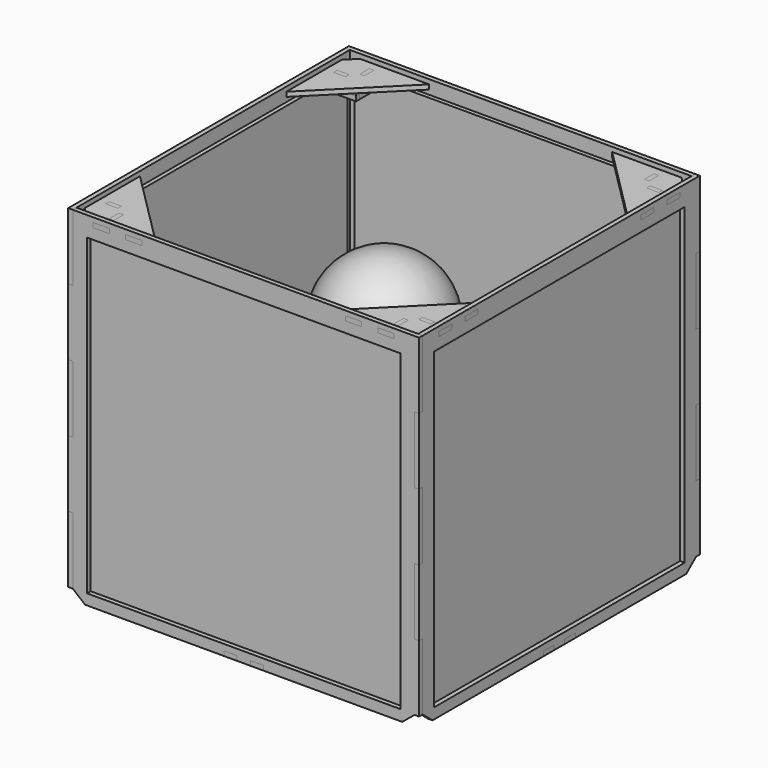
from build123d import *

# Parameters (mm, degrees)
F3_R      = 16
F3_R_2    = 15
F4_DEPTH  = 2.25
F5_W      = 2.25
F5_H      = 6.9285714286
F6_DEPTH  = 38
F7_DEPTH  = 2.25
F8_W      = 2.25
F8_H      = 6.6
F8_W_2    = 6.5
F8_H_2    = 2.25
F9_DEPTH  = 2.25
F11_W     = 160
F11_H     = 160
F12_DEPTH = 2
F13_W     = 154
F13_H     = 154
F13_W_2   = 8
F13_H_2   = 2.25
F14_DEPTH = 2.25
F15_W     = 6
F15_H     = 2.25
F15_W_2   = 2.25
F15_H_2   = 6
F16_DEPTH = 2.25
F18_DEPTH = 2.25
F20_DEPTH = 2.25
F21_W     = 2.25
F21_H     = 6.5
F21_W_2   = 4
F21_H_2   = 2.25
F22_DEPTH = 2.25
F24_DEPTH = 2.25
F25_COUNT = 4


with BuildPart() as f2:
    # F1 (on Front) → F2 (revolve)
    with BuildSketch(Plane.XZ):
        with BuildLine():
            Line((0, 143), (0, 10))
            Line((0, 10), (10, 10))
            Line((10, 10), (11.5, 20))
            Line((11.5, 20), (12.5, 25))
            Line((12.5, 25), (12.5, 36))
            Line((12.5, 36), (16, 36))
            Line((16, 36), (16, 38))
            Line((16, 38), (14, 38))
            Line((14, 38), (14, 40.25))
            Line((14, 40.25), (17.5, 40.25))
            Line((17.5, 40.25), (15, 48.25))
            Line((15, 48.25), (14, 48.25))
            Line((14, 48.25), (14, 63))
            Line((14, 63), (20, 72))
            Line((20, 72), (20, 85))
            Line((20, 85), (24, 95))
            ThreePointArc((24, 95), (26.83281573, 126.416407865), (0, 143))
        make_face()
    revolve(axis=Axis((0, 0, 76.5), (0, 0, -1)))


with BuildPart() as f4:
    # F3 (on face) → F4 (new body)
    with BuildSketch(Plane.XY.offset(38)):
        Polygon((-10.3928571429, 22), (-17.3214285714, 22), (-17.3214285714, 24.25), (-24.25, 24.25), (-24.25, 17.3214285714), (-22, 17.3214285714), (-22, 10.3928571429), (-24.25, 10.3928571429), (-24.25, 3.4642857143), (-22, 3.4642857143), (-22, -3.4642857143), (-24.25, -3.4642857143), (-24.25, -10.3928571429), (-22, -10.3928571429), (-22, -17.3214285714), (-24.25, -17.3214285714), (-24.25, -24.25), (-17.3214285714, -24.25), (-17.3214285714, -22), (-10.3928571429, -22), (-10.3928571429, -24.25), (-3.4642857143, -24.25), (-3.4642857143, -22), (3.4642857143, -22), (3.4642857143, -24.25), (10.3928571429, -24.25), (10.3928571429, -22), (17.3214285714, -22), (17.3214285714, -24.25), (24.25, -24.25), (24.25, -17.3214285714), (22, -17.3214285714), (22, -10.3928571429), (24.25, -10.3928571429), (24.25, -3.4642857143), (22, -3.4642857143), (22, 3.4642857143), (24.25, 3.4642857143), (24.25, 10.3928571429), (22, 10.3928571429), (22, 17.3214285714), (24.25, 17.3214285714), (24.25, 24.25), (17.3214285714, 24.25), (17.3214285714, 22), (10.3928571429, 22), (10.3928571429, 24.25), (3.4642857143, 24.25), (3.4642857143, 22), (-3.4642857143, 22), (-3.4642857143, 24.25), (-10.3928571429, 24.25), align=None)
        Circle(F3_R, mode=Mode.SUBTRACT)
        Circle(F3_R)
        Circle(F3_R_2, mode=Mode.SUBTRACT)
    extrude(amount=F4_DEPTH)


with BuildPart() as f6:
    # F5 (on face) → F6 (new body, through all)
    with BuildSketch(Plane(origin=(0, 0, 38), x_dir=(1, 0, 0), z_dir=(0, 0, -1))):
        with Locations((-23.125, 20.7857142857)):
            Rectangle(F5_W, F5_H)
        with Locations((-23.125, 13.8571428571)):
            Rectangle(F5_W, F5_H)
        with Locations((-23.125, 6.9285714286)):
            Rectangle(F5_W, F5_H)
        with Locations((-23.125, 0)):
            Rectangle(F5_W, F5_H)
        with Locations((-23.125, -6.9285714286)):
            Rectangle(F5_W, F5_H)
        with Locations((-23.125, -13.8571428571)):
            Rectangle(F5_W, F5_H)
        with Locations((-23.125, -20.7857142857)):
            Rectangle(F5_W, F5_H)
    extrude(amount=F6_DEPTH)

    # F5 (on face) → F7 (join, through all)
    with BuildSketch(Plane(origin=(0, 0, 38), x_dir=(1, 0, 0), z_dir=(0, 0, -1))):
        with Locations((-23.125, -13.8571428571)):
            Rectangle(F5_W, F5_H)
        with Locations((-23.125, 0)):
            Rectangle(F5_W, F5_H)
        with Locations((-23.125, 13.8571428571)):
            Rectangle(F5_W, F5_H)
    extrude(amount=-F7_DEPTH)

    # F8 (on face) → F9 (cut, through all)
    with BuildSketch(Plane(origin=(-24.25, 0, 0), x_dir=(0, -1, 0), z_dir=(-1, 0, 0))):
        Polygon((-24.25, 5), (-24.25, 0), (-9.75, 0), (-9.75, 2.25), (-16.25, 2.25), (-16.25, 5), align=None)
        Polygon((9.75, 0), (24.25, 0), (24.25, 5), (24.25, 11.6), (22, 11.6), (22, 5), (16.25, 5), (16.25, 2.25), (9.75, 2.25), align=None)
        with Locations((-23.125, 28.1)):
            Rectangle(F8_W, F8_H)
        with Locations((-23.125, 14.9)):
            Rectangle(F8_W, F8_H)
        with Locations((23.125, 34.7)):
            Rectangle(F8_W, F8_H)
        with Locations((23.125, 21.5)):
            Rectangle(F8_W, F8_H)
        with Locations((0, 1.125)):
            Rectangle(F8_W_2, F8_H_2)
    extrude(amount=-F9_DEPTH, mode=Mode.SUBTRACT)


with BuildPart() as f12:
    # F11 (on offset) → F12 (new body)
    with BuildSketch(Plane.YZ.offset(-82)):
        with Locations((0, 82.25)):
            Rectangle(F11_W, F11_H)
    extrude(amount=-F12_DEPTH)


with BuildPart() as f14:
    # F13 (on face) → F14 (new body)
    with BuildSketch(Plane(origin=(-84, 0, 0), x_dir=(0, -1, 0), z_dir=(-1, 0, 0))):
        Polygon((-84, 136.2), (-86.25, 136.2), (-86.25, 103.4), (-84, 103.4), (-84, 70.6), (-86.25, 70.6), (-86.25, 37.8), (-84, 37.8), (-84, 5), (-78, 0), (-9.75, 0), (-9.75, 2.25), (-3.25, 2.25), (-3.25, 0), (3.25, 0), (3.25, 2.25), (9.75, 2.25), (9.75, 0), (78, 0), (84, 5), (86.25, 5), (86.25, 37.8), (84, 37.8), (84, 70.6), (86.25, 70.6), (86.25, 103.4), (84, 103.4), (84, 136.2), (86.25, 136.2), (86.25, 169), (-84, 169), align=None)
        with Locations((0, 82.25)):
            Rectangle(F13_W, F13_H, mode=Mode.SUBTRACT)
        with Locations((-70, 165.625)):
            Rectangle(F13_W_2, F13_H_2, mode=Mode.SUBTRACT)
        with Locations((-54, 165.625)):
            Rectangle(F13_W_2, F13_H_2, mode=Mode.SUBTRACT)
        with Locations((54, 165.625)):
            Rectangle(F13_W_2, F13_H_2, mode=Mode.SUBTRACT)
        with Locations((70, 165.625)):
            Rectangle(F13_W_2, F13_H_2, mode=Mode.SUBTRACT)
    extrude(amount=F14_DEPTH)


with BuildPart() as f16:
    # F15 (on face) → F16 (new body, through all)
    with BuildSketch(Plane.XY.offset(164.5)):
        Polygon((-84, 74), (-86.25, 74), (-86.25, 66), (-84, 66), (-84, 58), (-86.25, 58), (-86.25, 50), (-84, 50), (-84, 45), (-45, 84), (-50, 84), (-50, 86.25), (-58, 86.25), (-58, 84), (-66, 84), (-66, 86.25), (-74, 86.25), (-74, 84), (-79, 84), (-84, 79), align=None)
        with Locations((-77, 70)):
            Rectangle(F15_W, F15_H, mode=Mode.SUBTRACT)
        with Locations((-70, 77)):
            Rectangle(F15_W_2, F15_H_2, mode=Mode.SUBTRACT)
    extrude(amount=F16_DEPTH)


with BuildPart() as f18:
    # F17 (on face) → F18 (new body, through all)
    with BuildSketch(Plane.XZ.offset(-71.125)):
        Polygon((-74, 166.75), (-80, 166.75), (-80, 164.5), (-82, 164.5), (-82, 157.75), (-68.875, 157.75), (-68.875, 160), (-71.125, 160), (-71.125, 162.25), (-68.875, 162.25), (-68.875, 164.5), (-74, 164.5), align=None)
    extrude(amount=F18_DEPTH)


with BuildPart() as f20:
    # F19 (on face) → F20 (new body, through all)
    with BuildSketch(Plane.YZ.offset(-71.125)):
        Polygon((80, 164.5), (80, 166.75), (74, 166.75), (74, 164.5), (71.125, 164.5), (71.125, 162.25), (68.8749999992, 162.25), (68.875, 160), (71.1249999993, 160), (71.125, 157.75), (82, 157.75), (82, 164.5), align=None)
    extrude(amount=F20_DEPTH)


with BuildPart() as f22:
    # F21 (on Top) → F22 (new body)
    with BuildSketch(Plane.XY):
        Polygon((-22, 16.25), (-84, 16.25), (-84, 9.75), (-86.25, 9.75), (-86.25, 3.25), (-84, 3.25), (-84, -3.25), (-86.25, -3.25), (-86.25, -9.75), (-84, -9.75), (-84, -16.25), (-22, -16.25), (-12.3743686708, -12.3743686708), (-10.2530483272, -10.2530483272), (-8.6620580695, -11.8440385849), (-4.0658639918, -7.2478445072), (-5.6568542495, -5.6568542495), (0, 0), (-5.6568542495, 5.6568542495), (-7.2478445072, 4.0658639918), (-11.8440385849, 8.6620580695), (-10.2530483272, 10.2530483272), (-12.3743686708, 12.3743686708), align=None)
        with Locations((-23.125, -6.5)):
            Rectangle(F21_W, F21_H, mode=Mode.SUBTRACT)
        with Locations((-76, 0)):
            Rectangle(F21_W_2, F21_H_2, mode=Mode.SUBTRACT)
        with Locations((-68, 0)):
            Rectangle(F21_W_2, F21_H_2, mode=Mode.SUBTRACT)
        with Locations((-23.125, 6.5)):
            Rectangle(F21_W, F21_H, mode=Mode.SUBTRACT)
    extrude(amount=F22_DEPTH)


with BuildPart() as f24:
    # F23 (on face) → F24 (new body, through all)
    with BuildSketch(Plane.XZ.offset(-1.125)):
        Polygon((-82, 2.25), (-78, 2.25), (-78, 0), (-74, 0), (-74, 2.25), (-70, 2.25), (-70, 0), (-66, 0), (-66, 2.25), (-62, 2.25), (-62, 6.25), (-82, 6.25), align=None)
    extrude(amount=F24_DEPTH)


with BuildPart() as f25_1:
    # F25: instance of F6
    add(f6.part.rotate(Axis((0, 0, 76.5), (0, 0, -1)), 1 * 360 / F25_COUNT))


with BuildPart() as f25_2:
    # F25: instance of F6
    add(f6.part.rotate(Axis((0, 0, 76.5), (0, 0, -1)), 2 * 360 / F25_COUNT))


with BuildPart() as f25_3:
    # F25: instance of F6
    add(f6.part.rotate(Axis((0, 0, 76.5), (0, 0, -1)), 3 * 360 / F25_COUNT))


with BuildPart() as f25_4:
    # F25: instance of F22
    add(f22.part.rotate(Axis((0, 0, 76.5), (0, 0, -1)), 1 * 360 / F25_COUNT))


with BuildPart() as f25_5:
    # F25: instance of F22
    add(f22.part.rotate(Axis((0, 0, 76.5), (0, 0, -1)), 2 * 360 / F25_COUNT))


with BuildPart() as f25_6:
    # F25: instance of F22
    add(f22.part.rotate(Axis((0, 0, 76.5), (0, 0, -1)), 3 * 360 / F25_COUNT))


with BuildPart() as f25_7:
    # F25: instance of F12
    add(f12.part.rotate(Axis((0, 0, 76.5), (0, 0, -1)), 1 * 360 / F25_COUNT))


with BuildPart() as f25_8:
    # F25: instance of F12
    add(f12.part.rotate(Axis((0, 0, 76.5), (0, 0, -1)), 2 * 360 / F25_COUNT))


with BuildPart() as f25_9:
    # F25: instance of F12
    add(f12.part.rotate(Axis((0, 0, 76.5), (0, 0, -1)), 3 * 360 / F25_COUNT))


with BuildPart() as f25_10:
    # F25: instance of F14
    add(f14.part.rotate(Axis((0, 0, 76.5), (0, 0, -1)), 1 * 360 / F25_COUNT))


with BuildPart() as f25_11:
    # F25: instance of F14
    add(f14.part.rotate(Axis((0, 0, 76.5), (0, 0, -1)), 2 * 360 / F25_COUNT))


with BuildPart() as f25_12:
    # F25: instance of F14
    add(f14.part.rotate(Axis((0, 0, 76.5), (0, 0, -1)), 3 * 360 / F25_COUNT))


with BuildPart() as f25_13:
    # F25: instance of F16
    add(f16.part.rotate(Axis((0, 0, 76.5), (0, 0, -1)), 1 * 360 / F25_COUNT))


with BuildPart() as f25_14:
    # F25: instance of F16
    add(f16.part.rotate(Axis((0, 0, 76.5), (0, 0, -1)), 2 * 360 / F25_COUNT))


with BuildPart() as f25_15:
    # F25: instance of F16
    add(f16.part.rotate(Axis((0, 0, 76.5), (0, 0, -1)), 3 * 360 / F25_COUNT))


with BuildPart() as f25_16:
    # F25: instance of F18
    add(f18.part.rotate(Axis((0, 0, 76.5), (0, 0, -1)), 1 * 360 / F25_COUNT))


with BuildPart() as f25_17:
    # F25: instance of F18
    add(f18.part.rotate(Axis((0, 0, 76.5), (0, 0, -1)), 2 * 360 / F25_COUNT))


with BuildPart() as f25_18:
    # F25: instance of F18
    add(f18.part.rotate(Axis((0, 0, 76.5), (0, 0, -1)), 3 * 360 / F25_COUNT))


with BuildPart() as f25_19:
    # F25: instance of F20
    add(f20.part.rotate(Axis((0, 0, 76.5), (0, 0, -1)), 1 * 360 / F25_COUNT))


with BuildPart() as f25_20:
    # F25: instance of F20
    add(f20.part.rotate(Axis((0, 0, 76.5), (0, 0, -1)), 2 * 360 / F25_COUNT))


with BuildPart() as f25_21:
    # F25: instance of F20
    add(f20.part.rotate(Axis((0, 0, 76.5), (0, 0, -1)), 3 * 360 / F25_COUNT))


with BuildPart() as f25_22:
    # F25: instance of F24
    add(f24.part.rotate(Axis((0, 0, 76.5), (0, 0, -1)), 1 * 360 / F25_COUNT))


with BuildPart() as f25_23:
    # F25: instance of F24
    add(f24.part.rotate(Axis((0, 0, 76.5), (0, 0, -1)), 2 * 360 / F25_COUNT))


with BuildPart() as f25_24:
    # F25: instance of F24
    add(f24.part.rotate(Axis((0, 0, 76.5), (0, 0, -1)), 3 * 360 / F25_COUNT))


solid = Compound([f2.part, f4.part, f6.part, f12.part, f14.part, f16.part, f18.part, f20.part, f22.part, f24.part, f25_1.part, f25_2.part, f25_3.part, f25_4.part, f25_5.part, f25_6.part, f25_7.part, f25_8.part, f25_9.part, f25_10.part, f25_11.part, f25_12.part, f25_13.part, f25_14.part, f25_15.part, f25_16.part, f25_17.part, f25_18.part, f25_19.part, f25_20.part, f25_21.part, f25_22.part, f25_23.part, f25_24.part])
